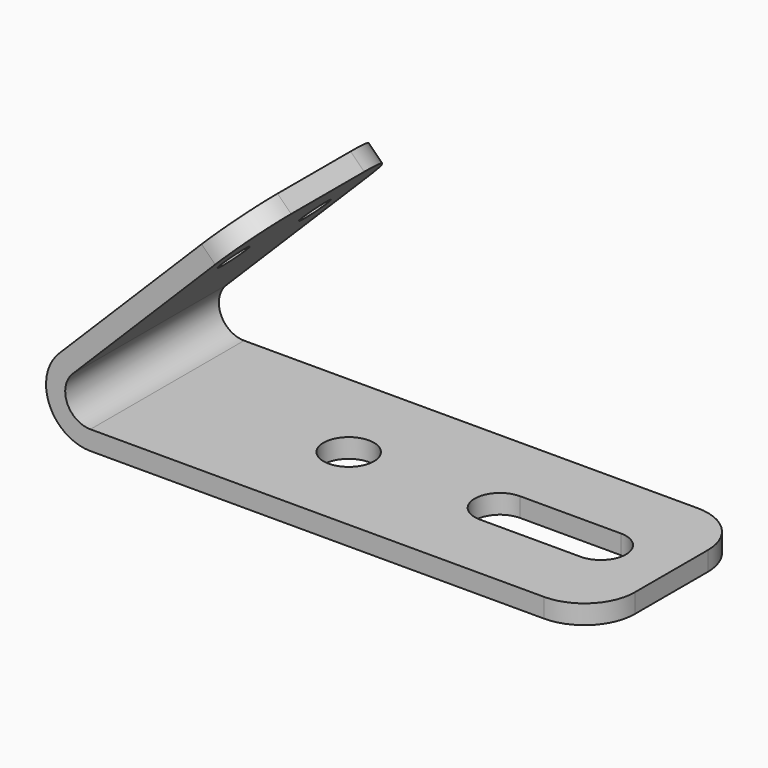
from build123d import *

# Parameters (mm, degrees)
F1_DEPTH = 9.525
F2_R     = 1.5
F3_DEPTH = 1.9
F4_R     = 2.5
F5_DEPTH = 1.9
F6_R     = 5
F7_R     = 5


# Not quite as in the source:
# - a pattern or mirror of a feature is missing from the dataset's text; its kind, count and spacing are read off the source's solid


with BuildPart() as f1:
    # F0 (on Front) → F1 (new body, symmetric)
    with BuildSketch(Plane.XZ):
        with BuildLine():
            Line((-50, 0), (0, 0))
            Line((0, 0), (0, 1.9))
            Line((0, 1.9), (-50, 1.9))
            ThreePointArc((-50, 1.9), (-52.3096988313, 3.4432914191), (-51.767766953, 6.167766953))
            Line((-51.767766953, 6.167766953), (-34.0900974233, 23.8454364826))
            Line((-34.0900974233, 23.8454364826), (-35.4336003076, 25.1889393669))
            Line((-35.4336003076, 25.1889393669), (-53.1112698372, 7.5112698372))
            ThreePointArc((-53.1112698372, 7.5112698372), (-54.065069943, 2.7161928976), (-50, 0))
        make_face()
    extrude(amount=F1_DEPTH, both=True)

    # F2 (on face) → F3 (cut, through all)
    with BuildSketch(Plane(origin=(-30.3112698372, 0, 30.3112698372), x_dir=(0, -1, 0), z_dir=(-0.7071067812, 0, 0.7071067812))):
        with Locations((5.025, -14.7440692221)):
            Circle(F2_R)
    f3 = extrude(amount=-F3_DEPTH, mode=Mode.SUBTRACT)

    # F3_copies: F3 across plane
    add(f3.mirror(Plane.ZX), mode=Mode.SUBTRACT)

    # F4 (on face) → F5 (cut, through all)
    with BuildSketch(Plane.XY.offset(1.9)):
        with BuildLine():
            Line((-17, -2.5), (-7, -2.5))
            ThreePointArc((-7, -2.5), (-4.5, 0), (-7, 2.5))
            Line((-7, 2.5), (-17, 2.5))
            ThreePointArc((-17, 2.5), (-19.5, 0), (-17, -2.5))
        make_face()
        with Locations((-32, 0)):
            Circle(F4_R)
    extrude(amount=-F5_DEPTH, mode=Mode.SUBTRACT)

    # F6
    f6_edges = [f1.edges().sort_by_distance(p)[0] for p in [
        (0, -9.525, 0.95),
        (0, 9.525, 0.95),
    ]]
    fillet(f6_edges, radius=F6_R)

    # F7
    f7_edges = [f1.edges().sort_by_distance(p)[0] for p in [
        (-34.761849, -9.525, 24.517188),
        (-34.761849, 9.525, 24.517188),
    ]]
    fillet(f7_edges, radius=F7_R)


solid = f1.part
